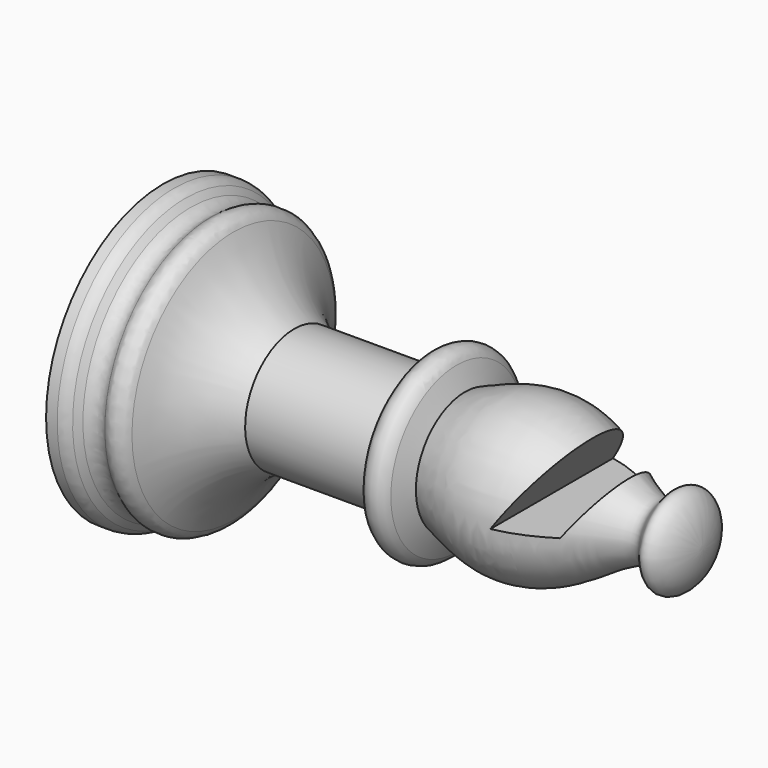
from build123d import *

# Parameters (mm, degrees)
F2_R     = 0.508
F4_DEPTH = 12.7


# Not quite as in the source:
# - a feature names something its author has since deleted; it is built from what else it names


with BuildPart() as f1:
    # F0 (on Front) → F1 (revolve)
    with BuildSketch(Plane.XZ):
        with BuildLine():
            Line((-19.05, 0), (0, 0))
            add(Edge.make_bspline(
                [(-8.3899357133, 2.1684124839), (-7.7378666571, 2.4291994979), (-6.3594848769, 2.9819840205), (-3.9352286815, 2.4825970716), (-1.4763863238, 0.40042843), (-0.9464125078, 2.1167979641), (0, 1.088525285), (0, 0)],
                knots=[0, 0, 0, 0, 0.208260679, 0.4391557931, 0.6719783024, 0.8051399106, 1, 1, 1, 1], degree=3))
            Line((-8.3899357133, 2.1684124839), (-9.1206210449, 3.9951248522))
            Line((-9.1206210449, 3.9951248522), (-9.9730862403, 2.1684124839))
            Line((-9.9730862403, 2.1684124839), (-14.4180862403, 2.1684124839))
            ThreePointArc((-14.4180862403, 2.1684124839), (-15.9392101959, 3.3955371388), (-16.7740837313, 5.1626362268))
            Line((-16.7740837313, 5.1626362268), (-17.7570101797, 4.3584250623))
            Line((-17.7570101797, 4.3584250623), (-18.415, 5.1626362268))
            Line((-18.415, 5.1626362268), (-19.05, 5.1626362268))
            Line((-19.05, 5.1626362268), (-19.05, 0))
        make_face()
    revolve(axis=Axis((-9.525, 0, 0), (-1, 0, 0)))

    # F2
    f2_edges = [f1.edges().sort_by_distance(p)[0] for p in [
        (-9.120621, 0, -3.995125),
        (-16.774084, 0, -5.162636),
        (-18.415, 0, -5.162636),
        (-17.75701, 0, -4.358425),
    ]]
    fillet(f2_edges, radius=F2_R)

    # F3 (on Front) → F4 (cut, symmetric)
    with BuildSketch(Plane.XZ):
        Polygon((-3.2252084929, 3.2164666336), (-5.3312126547, 0), (-3.4850692019, 0), (-1.9330305021, 2.3704040014), align=None)
    extrude(amount=F4_DEPTH, both=True, mode=Mode.SUBTRACT)


solid = f1.part
